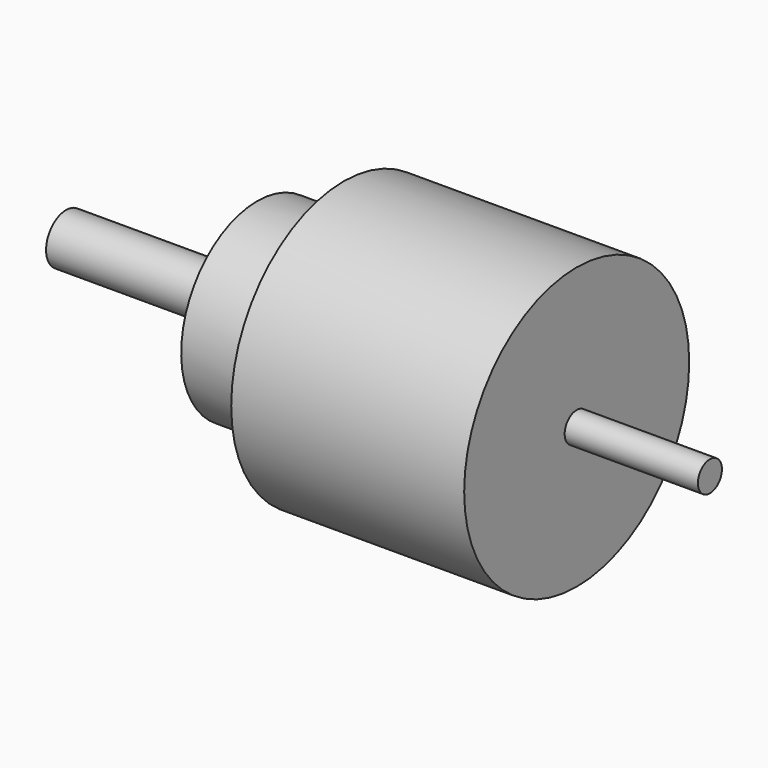
from build123d import *

# Parameters (mm, degrees)
F1_W = 13.31
F1_H = 1.5
F2_W = 41.21
F2_H = 1.5
F3_W = 19.1
F3_H = 2.5


with BuildPart() as f4:
    # F1 (on Front) → F4 (revolve)
    with BuildSketch(Plane.XZ):
        with Locations((6.655, 0.75)):
            Rectangle(F1_W, F1_H)
    revolve(axis=Axis((-18.85, 0, 0), (-1, 0, 0)))

    # F2 (on Front) → F5 (revolve)
    with BuildSketch(Plane.XZ):
        with Locations((-7.295, 0.75)):
            Rectangle(F2_W, F2_H)
    revolve(axis=Axis((-18.85, 0, 0), (-1, 0, 0)))


with BuildPart() as f4b:
    # F1 (on Front) → F4, piece 2 (revolve)
    with BuildSketch(Plane.XZ):
        Polygon((0, 14.05), (-23.2730562752, 14.05), (-25.9, 9.5), (-25.9, 1.5), (0, 1.5), align=None)
    revolve(axis=Axis((-18.85, 0, 0), (-1, 0, 0)))


with BuildPart() as f6:
    # F3 (on Front) → F6 (revolve)
    with BuildSketch(Plane.XZ):
        with Locations((-41.46, 1.25)):
            Rectangle(F3_W, F3_H)
        Polygon((-25.9, 9.5), (-31.91, 9.5), (-31.91, 2.5), (-31.91, 0), (-25.9, 0), align=None)
    revolve(axis=Axis((-18.85, 0, 0), (-1, 0, 0)))


solid = Compound([f4.part, f4b.part, f6.part])
